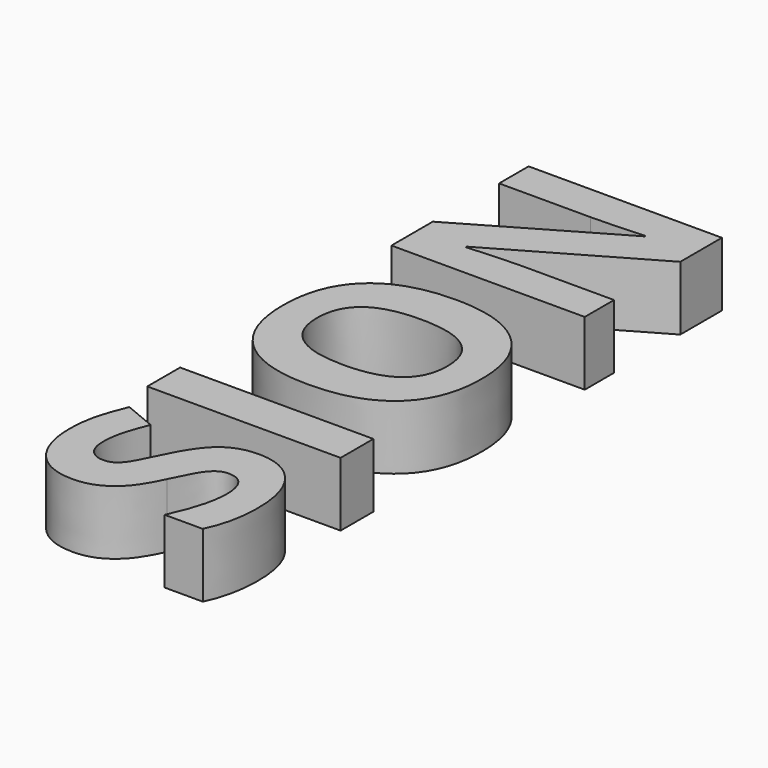
from build123d import *

# Parameters (mm, degrees)
F0_TEXT_SIZE = 8.450815868
F1_DEPTH     = 2


# Not quite as in the source:
# - Text() gives the source's letters only with a copy of the font that has no kerning and outlines rounded to 1/6400 em; it was checked with that copy


with BuildPart() as f1:
    # F0 (on Top) → F1 (new body)
    with BuildSketch(Plane.XY):
        with Locations(Location((-22.7264799178, -69.2818376701), (0, 0, 90))):
            Text('SION', F0_TEXT_SIZE, font='Open Sans', font_style=FontStyle.BOLD, text_align=(TextAlign.LEFT, TextAlign.BOTTOM))
    extrude(amount=F1_DEPTH)


solid = f1.part
